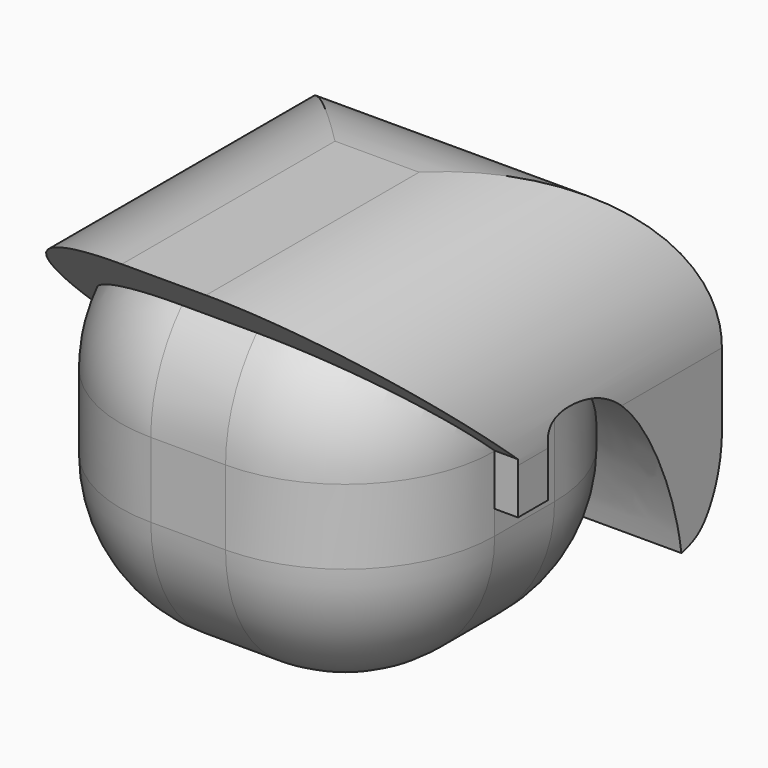
from build123d import *

# Parameters (mm, degrees)
F0_W          = 50.8
F0_H          = 50.8
F1_DEPTH      = 50.8
F2_R          = 20.32
F4_DEPTH      = 28.575
F4_DEPTH_BACK = 28.575
F5_T1_DEPTH   = 171.45
F5_T3_DEPTH   = 173.3631305569


# Not quite as in the source:
# - a fillet or chamfer that OpenCascade refuses, or shapes differently, is made with other operations: its cross-section is extruded or revolved along the edge and cut away or added


with BuildPart() as f1:
    # F0 (on Top) → F1 (new body)
    with BuildSketch(Plane.XY):
        Rectangle(F0_W, F0_H)
    extrude(amount=F1_DEPTH)

    # F2
    f2_edges = [f1.edges().sort_by_distance(p)[0] for p in [
        (0, 25.4, 50.8),
        (-25.4, 0, 50.8),
        (0, -25.4, 50.8),
        (25.4, 0, 50.8),
        (-25.4, 25.4, 25.4),
        (-25.4, -25.4, 25.4),
        (-25.4, 0, 0),
        (25.4, -25.4, 25.4),
        (0, -25.4, 0),
        (25.4, 25.4, 25.4),
        (25.4, 0, 0),
        (0, 25.4, 0),
    ]]
    fillet(f2_edges, radius=F2_R)

    # F3 (on Right) → F4 (join, two sides)
    with BuildSketch(Plane.YZ) as f4_sk:
        with BuildLine():
            Line((0, 23.585671559), (0, 30.6485332549))
            add(Edge.make_bspline(
                [(0, 30.6485332549), (0, 33.0861583352), (7.1330016043, 33.8045146668), (15.9690734978, 28.3277997784), (21.6986452978, 15.0790064451), (22.6556025445, 8.0415420234)],
                knots=[0, 0, 0, 0, 0.2426532196, 0.5552693869, 1, 1, 1, 1], degree=3))
            add(Edge.make_bspline(
                [(22.6556025445, 8.0415420234), (25.1164599813, 8.5749836186), (27.5161694097, 10.7134623968), (29.5368228108, 15.9953534603), (29.541708529, 20.0420022011)],
                knots=[0, 0, 0, 0, 0.4304337748, 1, 1, 1, 1], degree=3))
            Line((29.541708529, 20.0420022011), (29.541708529, 52.6639260352))
            Line((29.541708529, 52.6639260352), (-29.5214220279, 52.6639260352))
            Line((-29.5214220279, 52.6639260352), (-5.094319582, 30.5475965142))
            Line((-5.094319582, 30.5475965142), (-5.094319582, 23.585671559))
            Line((-5.094319582, 23.585671559), (0, 23.585671559))
        make_face()
    extrude(amount=F4_DEPTH)
    extrude(f4_sk.sketch, amount=-F4_DEPTH_BACK)

    # F5: fillet of radius 22.86 on 3 edges, made by hand

    # F5_s2 → F5_t1 (cut)
    with BuildSketch(Plane.YZ.offset(-85.725)):
        with BuildLine():
            ThreePointArc((29.541708529, 29.8039260352), (22.8461695469, 45.9683870531), (6.681708529, 52.6639260352))
            Line((6.681708529, 52.6639260352), (29.541708529, 52.6639260352))
            Line((29.541708529, 52.6639260352), (29.541708529, 29.8039260352))
        make_face()
    extrude(amount=F5_T1_DEPTH, mode=Mode.SUBTRACT)

    # F5_s4 → F5_t3 (cut)
    with BuildSketch(Plane.XZ.offset(-86.691708529)):
        with BuildLine():
            ThreePointArc((-28.575, 29.8039260352), (-21.8794610179, 45.9683870531), (-5.715, 52.6639260352))
            Line((-5.715, 52.6639260352), (-28.575, 52.6639260352))
            Line((-28.575, 52.6639260352), (-28.575, 29.8039260352))
        make_face()
        with BuildLine():
            ThreePointArc((28.575, 29.8039260352), (21.8794610179, 45.9683870531), (5.715, 52.6639260352))
            Line((5.715, 52.6639260352), (28.575, 52.6639260352))
            Line((28.575, 52.6639260352), (28.575, 29.8039260352))
        make_face()
    extrude(amount=F5_T3_DEPTH, mode=Mode.SUBTRACT)


solid = f1.part
